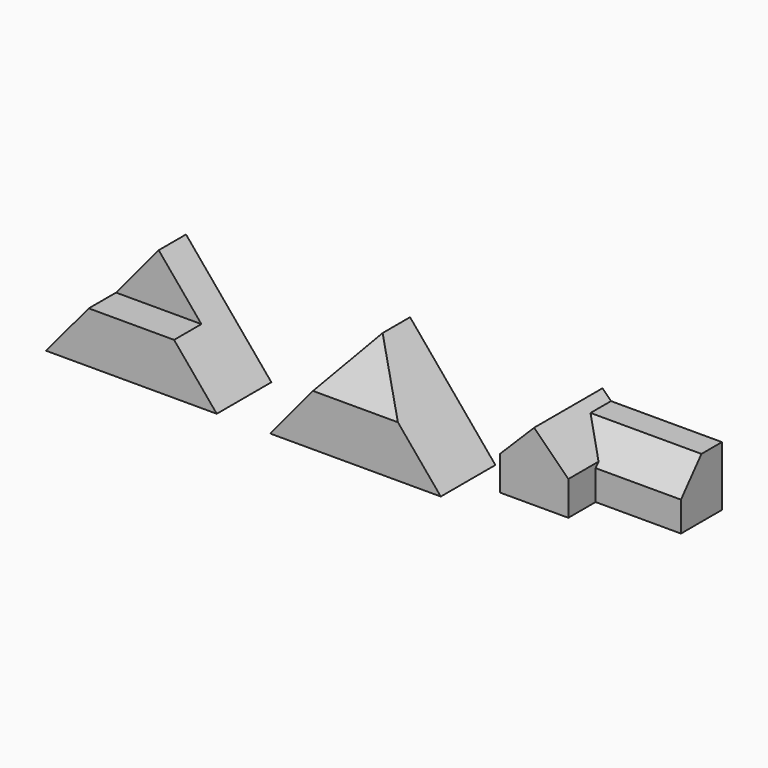
from build123d import *

# Parameters (mm, degrees)
F1_DEPTH       = 50.8
F3_DEPTH       = 50.8
F5_DEPTH       = 101.6
F8_DEPTH       = 239.522
F10_DEPTH      = 50.8
F10_DEPTH_BACK = 76.2
F9_W           = 127
F9_H           = 50.8
F11_DEPTH      = 76.2
F12_DEPTH      = 76.2
F14_DEPTH      = 167.386


with BuildPart() as f1:
    # F0 (on Front) → F1 (new body)
    with BuildSketch(Plane.XZ):
        Polygon((-127, 0), (0, 0), (-127, 152.4), align=None)
        Polygon((-254, 0), (-127, 0), (-127, 152.4), align=None)
    extrude(amount=F1_DEPTH)

    # F2 (on face) → F3 (join)
    with BuildSketch(Plane.XZ.offset(50.8)):
        Polygon((-190.5, 76.2), (-254, 0), (-127, 0), (-127, 76.2), align=None)
        Polygon((-127, 76.2), (-127, 0), (0, 0), (-63.5, 76.2), align=None)
    extrude(amount=F3_DEPTH)


with BuildPart() as f5:
    # F4 (on Front) → F5 (new body)
    with BuildSketch(Plane.XZ):
        Polygon((206.3964341254, 152.4), (79.3964341254, 0), (206.3964341254, 0), align=None)
        Polygon((206.3964341254, 152.4), (206.3964341254, 0), (333.3964341254, 0), align=None)
    extrude(amount=F5_DEPTH)

    # F7 (on offset) → F8 (cut)
    with BuildSketch(Plane.YZ.offset(342.138)):
        Polygon((-51.0394626021, 152.4), (-101.8394626021, 152.4), (-101.8394626021, 76.2), align=None)
    extrude(amount=-F8_DEPTH, mode=Mode.SUBTRACT)


with BuildPart() as f10:
    # F9 (on Front) → F10 (new body, two sides)
    with BuildSketch(Plane.XZ) as f10_sk:
        Polygon((380.9625402625, 50.8), (380.9625402625, 0), (431.7625402625, 0), (482.5625402625, 0), (482.5625402625, 50.8), (444.4625402625, 88.9), (431.7625402625, 101.6), align=None)
    extrude(amount=F10_DEPTH)
    extrude(f10_sk.sketch, amount=-F10_DEPTH_BACK)


with BuildPart() as f11:
    # F9 (on Front) → F11 (new body)
    with BuildSketch(Plane.XZ):
        with Locations((546.0625402625, 25.4)):
            Rectangle(F9_W, F9_H)
    extrude(amount=-F11_DEPTH)

    # F9 (on Front) → F12 (join)
    with BuildSketch(Plane.XZ):
        Polygon((444.4625402625, 88.9), (482.5625402625, 50.8), (609.5625402625, 50.8), (609.5625402625, 88.9), align=None)
    extrude(amount=-F12_DEPTH)

    # F13 (on face) → F14 (cut)
    with BuildSketch(Plane.YZ.offset(609.5625402625)):
        Polygon((0, 88.9), (0, 44.45), (38.1, 88.9), align=None)
    extrude(amount=-F14_DEPTH, mode=Mode.SUBTRACT)


solid = Compound([f1.part, f5.part, f10.part, f11.part])
